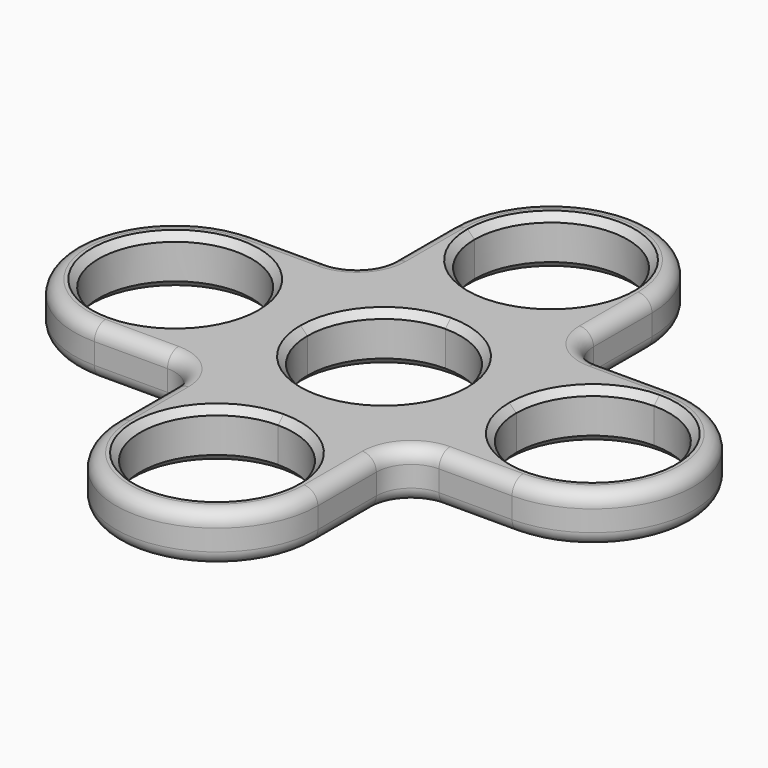
from build123d import *

# Parameters (mm, degrees)
F1_DEPTH = 7
F3_DEPTH = 7.001
F5_COUNT = 4
F7_R     = 5
F8_R     = 2
F9_SIZE  = 1


# Not quite as in the source:
# - a feature names something its author has since deleted; it is built from what else it names


with BuildPart() as f1:
    # F0 (on Top) → F1 (new body)
    with BuildSketch(Plane.XY):
        with BuildLine():
            ThreePointArc((-14.5, 0), (0, -14.5), (14.5, 0))
            ThreePointArc((14.5, 0), (0, 14.5), (-14.5, 0))
        make_face()
        with BuildLine():
            Line((14.5, -30), (14.5, 0))
            ThreePointArc((14.5, 0), (0, -14.5), (-14.5, 0))
            Line((-14.5, 0), (-14.5, -30))
            ThreePointArc((-14.5, -30), (0, -15.5), (14.5, -30))
        make_face()
        with BuildLine():
            ThreePointArc((-14.5, -30), (0, -44.5), (14.5, -30))
            ThreePointArc((14.5, -30), (0, -15.5), (-14.5, -30))
        make_face()
    extrude(amount=F1_DEPTH)

    # F2 (on face) → F3 (cut, through all)
    with BuildSketch(Plane.XY.offset(7)):
        with BuildLine():
            ThreePointArc((0, -11), (7.7781745931, -7.7781745931), (11, 0))
            ThreePointArc((11, 0), (-7.7781745931, 7.7781745931), (0, -11))
        make_face()
        with BuildLine():
            ThreePointArc((11, -30), (7.7781745931, -22.2218254069), (0, -19))
            ThreePointArc((0, -19), (-7.7781745931, -37.7781745931), (11, -30))
        make_face()
    extrude(amount=-F3_DEPTH, mode=Mode.SUBTRACT)


with BuildPart() as f5_1:
    # F5: instance of F1
    add(f1.part.rotate(Axis((0, 0, 13.2415927947), (0, 0, 1)), 1 * 360 / F5_COUNT))


with BuildPart() as f5_2:
    # F5: instance of F1
    add(f1.part.rotate(Axis((0, 0, 13.2415927947), (0, 0, 1)), 2 * 360 / F5_COUNT))


with BuildPart() as f5_3:
    # F5: instance of F1
    add(f1.part.rotate(Axis((0, 0, 13.2415927947), (0, 0, 1)), 3 * 360 / F5_COUNT))


with BuildPart() as f1_1:
    add(f1.part)

    # F6: union F5_3, F5_2, F5_1
    add(f5_3.part)
    add(f5_2.part)
    add(f5_1.part)

    # F7
    f7_edges = [f1_1.edges().sort_by_distance(p)[0] for p in [
        (14.5, -14.5, 3.5),
        (14.5, 14.5, 3.5),
        (-14.5, -14.5, 3.5),
        (-14.5, 14.5, 3.5),
    ]]
    fillet(f7_edges, radius=F7_R)

    # F8
    f8_edges = [f1_1.edges().sort_by_distance(p)[0] for p in [
        (44.5, 0, 7),
        (0, -44.5, 0),
        (24.75, -14.5, 0),
        (15.964466, -15.964466, 0),
        (44.5, 0, 0),
        (14.5, -24.75, 0),
        (24.75, 14.5, 0),
        (15.964466, 15.964466, 0),
        (-14.5, -24.75, 0),
        (14.5, 24.75, 0),
        (-15.964466, -15.964466, 0),
        (0, 44.5, 0),
        (-24.75, -14.5, 0),
        (-14.5, 24.75, 0),
        (-44.5, 0, 0),
        (-15.964466, 15.964466, 0),
        (-24.75, 14.5, 0),
        (24.75, -14.5, 7),
        (15.964466, -15.964466, 7),
        (14.5, -24.75, 7),
        (24.75, 14.5, 7),
        (0, -44.5, 7),
        (15.964466, 15.964466, 7),
        (-14.5, -24.75, 7),
        (14.5, 24.75, 7),
        (-15.964466, -15.964466, 7),
        (0, 44.5, 7),
        (-24.75, -14.5, 7),
        (-14.5, 24.75, 7),
        (-44.5, 0, 7),
        (-15.964466, 15.964466, 7),
        (-24.75, 14.5, 7),
    ]]
    fillet(f8_edges, radius=F8_R)

    # F9
    f9_edges = [f1_1.edges().sort_by_distance(p)[0] for p in [
        (0, 11, 7),
        (0, 41, 7),
        (-41, 0, 7),
        (0, -41, 7),
        (41, 0, 7),
        (0, -41, 0),
        (41, 0, 0),
        (0, 41, 0),
        (-41, 0, 0),
        (0, 11, 0),
    ]]
    chamfer(f9_edges, length=F9_SIZE)


solid = f1_1.part
